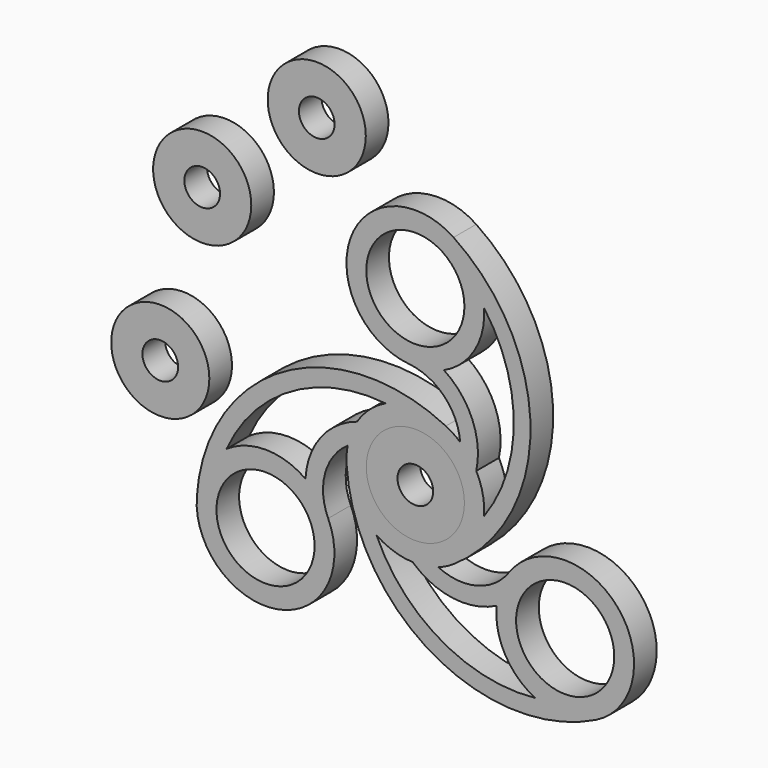
from build123d import *

# Parameters (mm, degrees)
F1_R     = 11
F2_DEPTH = 6.35
F3_COUNT = 3
F1_R_2   = 4
F4_DEPTH = 6.35
F5_R     = 11
F5_R_2   = 4
F6_DEPTH = 6.35
F7_DEPTH = 6.35
F8_DEPTH = 6.35


with BuildPart() as f2:
    # F1 (on Front) → F2 (new body)
    with BuildSketch(Plane.XZ):
        with BuildLine():
            ThreePointArc((-1.4612667351, 23.4131014427), (6.4162478072, 19.6674691464), (10.0427237927, 11.7343947997))
            ThreePointArc((10.0427237927, 11.7343947997), (-15.4174391876, 0.9246033691), (8.5683350764, -12.850523589))
            ThreePointArc((8.5683350764, -12.850523589), (25.8238631569, 19.3944799292), (8.5683350764, 51.6394834474))
            ThreePointArc((8.5683350764, 51.6394834474), (-14.5536856284, 43.9602804945), (-1.4612667351, 23.4131014427))
        make_face()
        Circle(F1_R, mode=Mode.SUBTRACT)
        with Locations((0, 38.7889598584)):
            Circle(F1_R, mode=Mode.SUBTRACT)
        with BuildLine():
            ThreePointArc((13.6634637034, 7.2015333173), (12.7718103509, 17.0994927213), (6.4162478072, 24.7396151559))
            ThreePointArc((6.4162478072, 24.7396151559), (13.3011693847, 30.9384047512), (15.4005525832, 39.9616928305))
            ThreePointArc((15.4005525832, 39.9616928305), (22.0786916612, 19.3944799292), (15.4005525832, -1.1727329721))
            ThreePointArc((15.4005525832, -1.1727329721), (15.1232055017, 3.1370332871), (13.6634637034, 7.2015333173))
        make_face(mode=Mode.SUBTRACT)
    extrude(amount=F2_DEPTH)

    # F3: F2 ×3 about axis
    f3_axis = Axis((0, -6.35, 0), (0, -1, 0))


with BuildPart() as f2_1:
    add(f2.part)
    for i in range(1, F3_COUNT):
        add(f2.part.rotate(f3_axis, i * 360 / F3_COUNT))


with BuildPart() as f4:
    # F1 (on Front) → F4 (new body)
    with BuildSketch(Plane.XZ):
        Circle(F1_R)
        Circle(F1_R_2, mode=Mode.SUBTRACT)
    extrude(amount=F4_DEPTH)


with BuildPart() as f6:
    # F5 (on Front) → F6 (new body)
    with BuildSketch(Plane.XZ):
        with Locations((-22.1062817913, 65.2865074809)):
            Circle(F5_R)
        with Locations((-22.1062817913, 65.2865074809)):
            Circle(F5_R_2, mode=Mode.SUBTRACT)
    extrude(amount=F6_DEPTH)


with BuildPart() as f7:
    # F5 (on Front) → F7 (new body)
    with BuildSketch(Plane.XZ):
        with Locations((-47.7854066729, 43.2241640761)):
            Circle(F5_R)
        with Locations((-47.7854066729, 43.2241640761)):
            Circle(F5_R_2, mode=Mode.SUBTRACT)
    extrude(amount=F7_DEPTH)


with BuildPart() as f8:
    # F5 (on Front) → F8 (new body)
    with BuildSketch(Plane.XZ):
        with Locations((-57.1890292476, 5.9713492778)):
            Circle(F5_R)
        with Locations((-57.1890292476, 5.9713492778)):
            Circle(F5_R_2, mode=Mode.SUBTRACT)
    extrude(amount=F8_DEPTH)


solid = Compound([f2_1.part, f4.part, f6.part, f7.part, f8.part])
